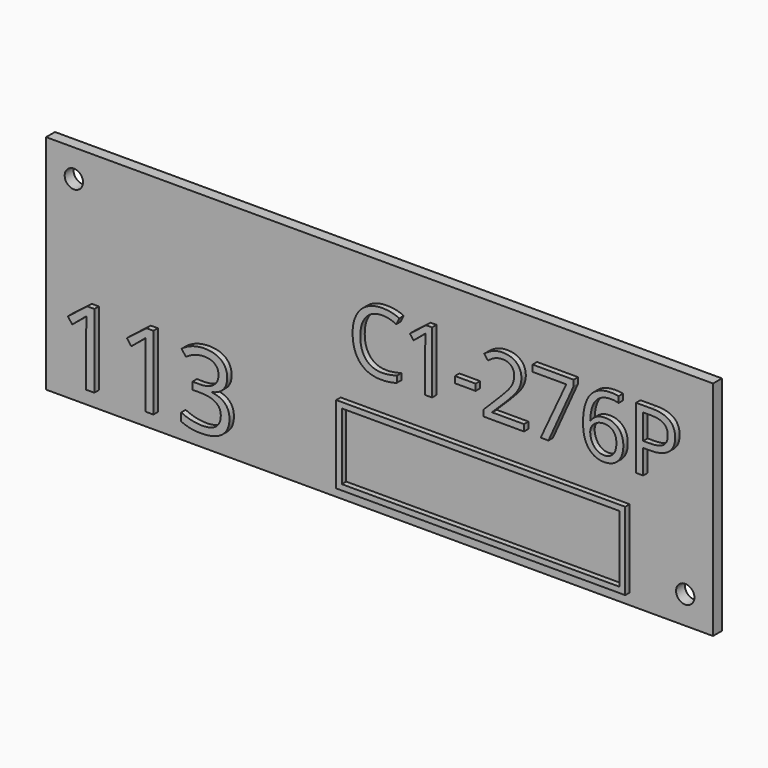
from build123d import *

# Parameters (mm, degrees)
F0_W         = 120
F0_H         = 40
F1_DEPTH     = 2
F3_D         = 3.3
F4_TEXT_SIZE = 15.5635715154
F5_DEPTH     = 1
F6_TEXT_SIZE = 18.5894526641
F7_DEPTH     = 1
F8_W         = 52
F8_H         = 14
F8_W_2       = 49.99999962
F8_H_2       = 11.99999962
F9_DEPTH     = 1


# Not quite as in the source:
# - Text() gives the source's letters only with a copy of the font that has no kerning and outlines rounded to 1/6400 em; it was checked with that copy


with BuildPart() as f1:
    # F0 (on Front) → F1 (new body)
    with BuildSketch(Plane.XZ):
        Rectangle(F0_W, F0_H)
    extrude(amount=F1_DEPTH)

    # F3 (through all)
    with Locations(Plane.XZ.offset(2)):
        with Locations((-55, 15), (55, -15)):
            Hole(F3_D / 2)

    # F4 (on face) → F5 (join)
    with BuildSketch(Plane.XZ.offset(2)):
        with Locations((-5, 2)):
            Text('C1-276P', F4_TEXT_SIZE, font='Open Sans', text_align=(TextAlign.LEFT, TextAlign.BOTTOM))
    extrude(amount=F5_DEPTH)

    # F6 (on face) → F7 (join)
    with BuildSketch(Plane.XZ.offset(2)):
        with Locations((-57, -17)):
            Text('113', F6_TEXT_SIZE, font='Open Sans', text_align=(TextAlign.LEFT, TextAlign.BOTTOM))
    extrude(amount=F7_DEPTH)

    # F8 (on face) → F9 (join)
    with BuildSketch(Plane.XZ.offset(2)):
        with Locations((19, -11)):
            Rectangle(F8_W, F8_H)
        with Locations((19, -11)):
            Rectangle(F8_W_2, F8_H_2, mode=Mode.SUBTRACT)
    extrude(amount=F9_DEPTH)


solid = f1.part
